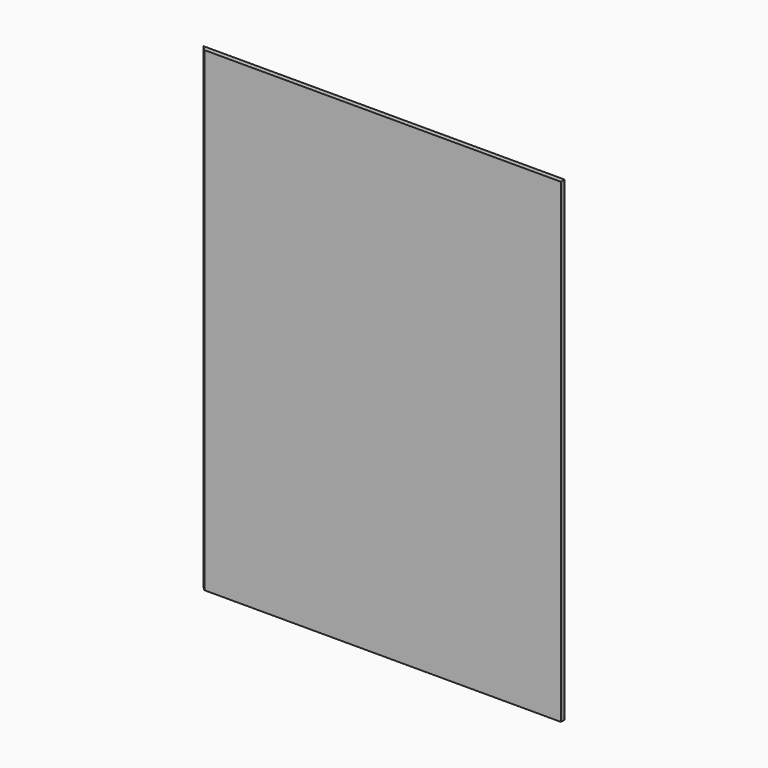
from build123d import *

# Parameters (mm, degrees)
F0_W        = 80
F0_H        = 100
F1_DEPTH    = 0.5
F2_T1_DEPTH = 125.7168298797


# Not quite as in the source:
# - a fillet or chamfer that OpenCascade refuses, or shapes differently, is made with other operations: its cross-section is extruded or revolved along the edge and cut away or added


with BuildPart() as f1:
    # F0 (on Front) → F1 (new body, symmetric)
    with BuildSketch(Plane.XZ):
        Rectangle(F0_W, F0_H)
    extrude(amount=F1_DEPTH, both=True)

    # F2: chamfer of 5 on 1 edges, made by hand

    # F2_s2 → F2_t1 (cut)
    with BuildSketch(Plane.XY.offset(-62.8584149398)):
        Polygon((-35, -0.5), (-40, 4.5), (-40, -0.5), align=None)
    extrude(amount=F2_T1_DEPTH, mode=Mode.SUBTRACT)


solid = f1.part
